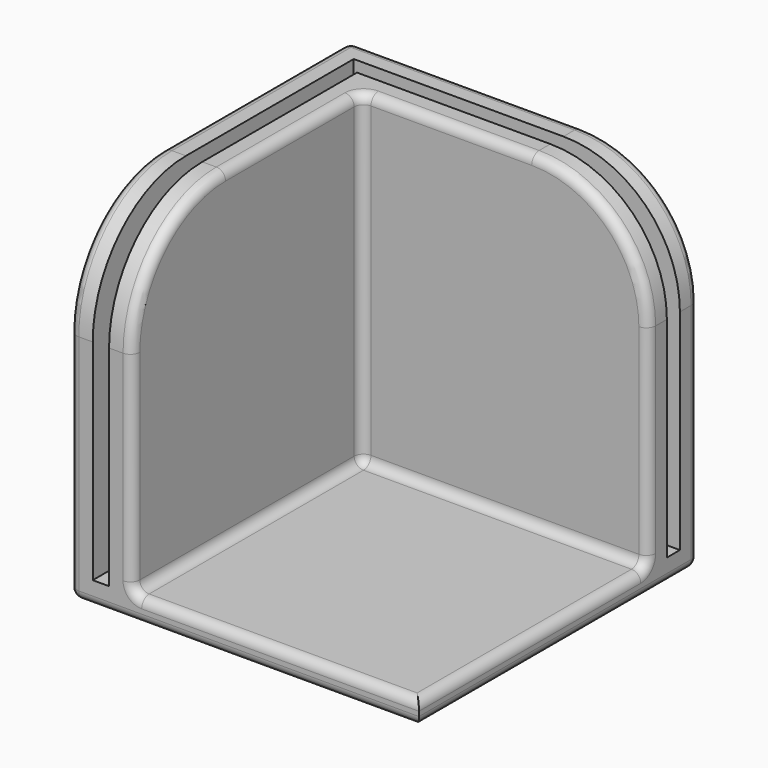
from build123d import *

# Parameters (mm, degrees)
F0_W     = 75
F0_H     = 75
F1_DEPTH = 5
F2_W     = 70
F2_H     = 5
F3_DEPTH = 70
F4_W     = 61.5
F4_H     = 5
F5_DEPTH = 70
F6_R     = 25
F7_R     = 2


with BuildPart() as f1:
    # F0 (on Top) → F1 (new body)
    with BuildSketch(Plane.XY):
        Rectangle(F0_W, F0_H)
    extrude(amount=F1_DEPTH)

    # F2 (on face) → F3 (join)
    with BuildSketch(Plane.XY.offset(5)):
        Polygon((-32.5, 37.5), (-37.5, 37.5), (-37.5, -37.5), (-32.5, -37.5), (-32.5, 32.5), align=None)
        with Locations((2.5, 35)):
            Rectangle(F2_W, F2_H)
    extrude(amount=F3_DEPTH)

    # F4 (on face) → F5 (join, through all)
    with BuildSketch(Plane.XY.offset(5)):
        Polygon((-29, 29), (-29, -37.5), (-24, -37.5), (-24, 24), (-24, 29), align=None)
        with Locations((6.75, 26.5)):
            Rectangle(F4_W, F4_H)
    extrude(amount=F5_DEPTH)

    # F6
    f6_edges = [f1.edges().sort_by_distance(p)[0] for p in [
        (-35, -37.5, 75),
        (-26.5, -37.5, 75),
        (37.5, 26.5, 75),
        (37.5, 35, 75),
    ]]
    fillet(f6_edges, radius=F6_R)

    # F7
    f7_edges = [f1.edges().sort_by_distance(p)[0] for p in [
        (37.5, 37.5, 25),
        (30.17767, 37.5, 67.67767),
        (0, 37.5, 0),
        (-12.5, 37.5, 75),
        (-37.5, 37.5, 37.5),
        (0, -37.5, 0),
        (37.5, 0, 0),
        (-37.5, 0, 0),
        (-37.5, 12.5, 75),
        (-37.5, -30.17767, 67.67767),
        (-37.5, -37.5, 25),
        (-24, -6.75, 5),
        (6.75, 24, 5),
        (37.5, -6.75, 5),
        (6.75, -37.5, 5),
        (-24, 24, 40),
        (-24, -37.5, 27.5),
        (37.5, 24, 27.5),
        (-24, -30.17767, 67.67767),
        (-24, 5.75, 75),
        (30.17767, 24, 67.67767),
        (-5.75, 24, 75),
    ]]
    fillet(f7_edges, radius=F7_R)


solid = f1.part
